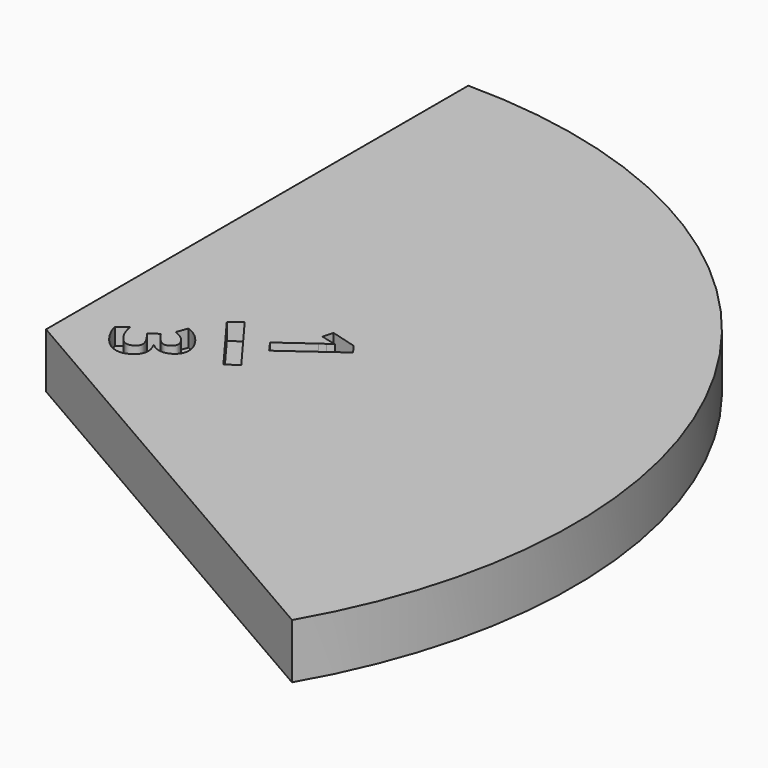
from build123d import *

# Parameters (mm, degrees)
F1_DEPTH     = 6.5
F2_R         = 12.5
F3_DEPTH     = 5
F4_TEXT_SIZE = 10.8747925081
F5_DEPTH     = 2
F7_DEPTH     = 2


# Not quite as in the source:
# - Text() gives the source's letters only with a copy of the font that has no kerning and outlines rounded to 1/6400 em; it was checked with that copy


with BuildPart() as f1:
    # F0 (on Top) → F1 (new body)
    with BuildSketch(Plane.XY):
        with BuildLine():
            Line((0, 0), (54.1265877365, -31.25))
            ThreePointArc((54.1265877365, -31.25), (54.1265877365, 31.25), (0, 62.5))
            Line((0, 62.5), (0, 0))
        make_face()
    extrude(amount=F1_DEPTH)

    # F2 (on face) → F3 (cut)
    with BuildSketch(Plane(origin=(0, 0, 0), x_dir=(1, 0, 0), z_dir=(0, 0, -1))):
        with Locations((45.6975325942, 7.2615263052)):
            Circle(F2_R)
        with Locations((40.6895875931, -22.7861702442)):
            Circle(F2_R)
        with Locations((16.6514292359, -42.8179651499)):
            Circle(F2_R)
    extrude(amount=-F3_DEPTH, mode=Mode.SUBTRACT)

    # F4 (on face) → F5 (cut)
    with BuildSketch(Plane.XY.offset(6.5)):
        with Locations(Location((16.1424053835, 13.1917312777), (0, 0, -54.12142949))):
            Text('1', F4_TEXT_SIZE, font='Open Sans', font_style=FontStyle.BOLD, text_align=(TextAlign.LEFT, TextAlign.BOTTOM))
        with Locations(Location((4.1588753793, 4.5239310049), (0, 0, -54.12142949))):
            Text('3', F4_TEXT_SIZE, font='Open Sans', font_style=FontStyle.BOLD, text_align=(TextAlign.LEFT, TextAlign.BOTTOM))
    extrude(amount=-F5_DEPTH, mode=Mode.SUBTRACT)

    # F6 (on face) → F7 (cut)
    with BuildSketch(Plane.XY.offset(6.5)):
        Polygon((13.4486613109, 12.5864416158), (12.1195421945, 11.6008027951), (17.2182662376, 4.7252501558), (18.547385354, 5.7108889765), align=None)
    extrude(amount=-F7_DEPTH, mode=Mode.SUBTRACT)


solid = f1.part
